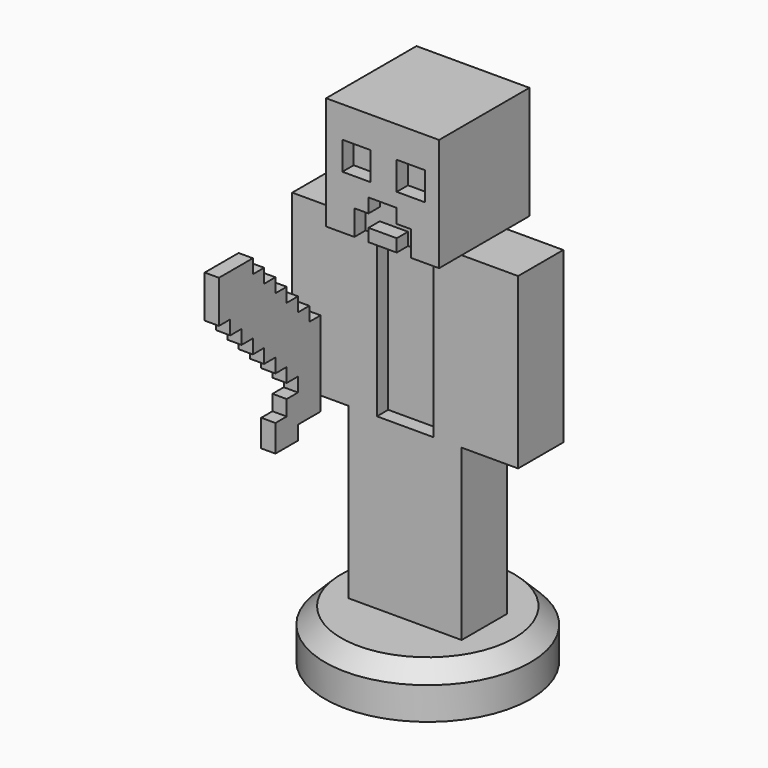
from build123d import *

# Parameters (mm, degrees)
F0_R      = 31.75
F1_DEPTH  = 15
F2_SIZE   = 5
F3_R      = 25
F4_DEPTH  = 10
F5_SIZE2  = 9.99999
F5_SIZE   = 24.99999
F6_W      = 34.925
F6_H      = 17.4625
F7_DEPTH  = 104.774
F10_W     = 34.925
F10_H     = 34.925
F11_DEPTH = 34.925
F12_W     = 17.4625
F12_H     = 17.4625
F13_DEPTH = 17.4625
F14_DEPTH = 34.925
F15_W     = 17.4625
F15_H     = 17.4625
F15_H_2   = 34.925
F16_DEPTH = 17.4625
F19_W     = 8.73125
F19_H     = 8.73125
F20_DEPTH = 4.365625
F17_W     = 4.365625
F17_H     = 4.365625
F23_DEPTH = 4.365625
F24_DEPTH = 4.365625
F25_W     = 4.4006995887
F25_H     = 4.365625
F26_DEPTH = 4.365625
F27_DEPTH = 8.73125
F28_W     = 4.4006995887
F28_H     = 4.365625
F29_DEPTH = 4.365625
F30_W     = 4.4006995887
F30_H     = 4.365625
F31_DEPTH = 4.365625
F32_W     = 4.4006995887
F32_H     = 4.365
F33_DEPTH = 4.365625
F34_DEPTH = 8.73125
F35_W     = 4.4006995887
F35_H     = 4.365
F36_DEPTH = 4.365625
F37_DEPTH = 8.73125
F38_W     = 4.4006995887
F38_H     = 4.365
F39_DEPTH = 4.365625
F40_DEPTH = 8.73125
F42_W     = 4.365625
F42_H     = 4.365625
F43_DEPTH = 4.365625
F44_DEPTH = 4.365625
F46_DEPTH = 8.73125
F47_W     = 4.365625
F47_H     = 4.365625
F48_DEPTH = 25
F41_W     = 4.4006995887
F41_H     = 4.365
F49_DEPTH = 4.365625
F50_DEPTH = 8.73125
F51_W     = 4.4006995887
F51_H     = 4.365
F52_DEPTH = 4.365625
F53_DEPTH = 8.73215
F54_W     = 4.4006995887
F54_H     = 4.3659
F55_DEPTH = 4.365625
F56_DEPTH = 4.365625
F57_W     = 4.4006995887
F57_H     = 4.365625
F58_DEPTH = 4.365625
F59_W     = 4.4006995887
F59_H     = 8.73125
F60_DEPTH = 4.365625
F61_DEPTH = 4.365625
F62_DEPTH = 4.365625
F63_DEPTH = 4.365625
F64_W     = 4.4006995887
F64_H     = 8.73125
F65_DEPTH = 4.365625
F66_W     = 4.4006995887
F66_H     = 4.36625
F66_H_2   = 4.365625
F67_DEPTH = 4.365625
F68_W     = 4.4006995887
F68_H     = 4.365625
F69_DEPTH = 4.365625
F70_W     = 4.4006995887
F70_H     = 4.4238492846
F70_H_2   = 3.9164990911
F71_DEPTH = 4.3565625
F21_W     = 17.4625
F21_H     = 52.3875
F72_DEPTH = 4.365625


# Not quite as in the source:
# - a fillet or chamfer is up to 0.001 mm smaller than in the source, because OpenCascade refuses the exact size


with BuildPart() as f1:
    # F0 (on Top) → F1 (new body)
    with BuildSketch(Plane.XY):
        Circle(F0_R)
    extrude(amount=F1_DEPTH)

    # F2
    f2_edges = [f1.edges().sort_by_distance(p)[0] for p in [
        (-31.75, 0, 15),
    ]]
    chamfer(f2_edges, length=F2_SIZE)

    # F3 (on face) → F4 (cut)
    with BuildSketch(Plane(origin=(0, 0, 0), x_dir=(1, 0, 0), z_dir=(0, 0, -1))):
        Circle(F3_R)
    extrude(amount=-F4_DEPTH, mode=Mode.SUBTRACT)

    # F5 (size 25 and 10 in the source; OpenCascade refuses exactly that, so slightly less here)
    f5_edges = [f1.edges().sort_by_distance(p)[0] for p in [
        (-25, 0, 10),
    ]]
    f5_side = f1.faces().sort_by_distance((0, 0, 10))[0]
    chamfer(f5_edges, length=F5_SIZE, length2=F5_SIZE2, reference=f5_side)

    # F6 (on face) → F7 (join)
    with BuildSketch(Plane.XY.offset(15)):
        Rectangle(F6_W, F6_H)
    extrude(amount=F7_DEPTH)

    # F10 (on face) → F11 (join)
    with BuildSketch(Plane.XY.offset(119.774)):
        Rectangle(F10_W, F10_H)
    extrude(amount=F11_DEPTH)

    # F12 (on face) → F13 (join)
    with BuildSketch(Plane.YZ.offset(17.4625)):
        with Locations((0, 111.04275)):
            Rectangle(F12_W, F12_H)
    extrude(amount=F13_DEPTH)

    # F14 (add): a face of the model
    f14_faces = [f1.faces().sort_by_distance(p)[0] for p in [
        (26.19375, 0, 102.3115),
    ]]
    extrude(f14_faces, amount=F14_DEPTH)

    # F15 (on face) → F16 (join)
    with BuildSketch(Plane(origin=(-17.4625, 0, 0), x_dir=(0, -1, 0), z_dir=(-1, 0, 0))):
        with Locations((0, 111.04275)):
            Rectangle(F15_W, F15_H)
        with Locations((0, 84.849)):
            Rectangle(F15_W, F15_H_2)
    extrude(amount=F16_DEPTH)

    # F19 (on face) → F20 (cut)
    with BuildSketch(Plane.XZ.offset(17.4625)):
        Polygon((-8.73125, 127.5853067636), (-8.73125, 119.774), (-4.365625, 119.774), (-4.365625, 123.6796533818), (4.365625, 123.6796533818), (4.365625, 119.774), (8.73125, 119.774), (8.73125, 127.5853067636), (4.365625, 127.5853067636), (4.365625, 131.9509317636), (-4.365625, 131.9509317636), (-4.365625, 127.5853067636), align=None)
        with Locations((-8.068405883, 140.6821817636)):
            Rectangle(F19_W, F19_H)
        with Locations((8.73125, 140.6821817636)):
            Rectangle(F19_W, F19_H)
    extrude(amount=-F20_DEPTH, mode=Mode.SUBTRACT)

    # F17 (on face) → F23 (join)
    with BuildSketch(Plane(origin=(0, 8.73125, 0), x_dir=(-1, 0, 0), z_dir=(0, 1, 0))):
        with Locations((28.3765625, 69.5693125)):
            Rectangle(F17_W, F17_H)
    extrude(amount=F23_DEPTH)

    # F24 (add): a face of the model
    f24_faces = [f1.faces().sort_by_distance(p)[0] for p in [
        (-28.3765625, 10.9140625, 71.752125),
    ]]
    extrude(f24_faces, amount=F24_DEPTH)

    # F25 (on face) → F26 (join)
    with BuildSketch(Plane.XZ.offset(8.73125)):
        with Locations((-28.3590252057, 69.5693125)):
            Rectangle(F25_W, F25_H)
    extrude(amount=F26_DEPTH)

    # F27 (add): a face of the model
    f27_faces = [f1.faces().sort_by_distance(p)[0] for p in [
        (-28.3590252057, -10.9140625, 71.752125),
    ]]
    extrude(f27_faces, amount=F27_DEPTH)

    # F28 (on face) → F29 (join)
    with BuildSketch(Plane.XZ.offset(13.096875)):
        with Locations((-28.3590252057, 73.9349375)):
            Rectangle(F28_W, F28_H)
        with Locations((-28.3590252057, 78.3005625)):
            Rectangle(F28_W, F28_H)
    extrude(amount=F29_DEPTH)

    # F30 (on face) → F31 (join)
    with BuildSketch(Plane.XY.offset(80.483375)):
        with Locations((-28.3590252057, -15.2796875)):
            Rectangle(F30_W, F30_H)
    extrude(amount=F31_DEPTH)

    # F32 (on face) → F33 (join)
    with BuildSketch(Plane.XZ.offset(17.4625)):
        with Locations((-28.3590252057, 78.300875)):
            Rectangle(F32_W, F32_H)
    extrude(amount=F33_DEPTH)

    # F34 (add): a face of the model
    f34_faces = [f1.faces().sort_by_distance(p)[0] for p in [
        (-28.3590252057, -19.6453125, 80.483375),
    ]]
    extrude(f34_faces, amount=F34_DEPTH)

    # F35 (on face) → F36 (join)
    with BuildSketch(Plane.XZ.offset(21.828125)):
        with Locations((-28.3590252057, 82.6665)):
            Rectangle(F35_W, F35_H)
    extrude(amount=F36_DEPTH)

    # F37 (add): a face of the model
    f37_faces = [f1.faces().sort_by_distance(p)[0] for p in [
        (-28.3590252057, -24.0109375, 84.849),
    ]]
    extrude(f37_faces, amount=F37_DEPTH)

    # F38 (on face) → F39 (join)
    with BuildSketch(Plane.XZ.offset(26.19375)):
        with Locations((-28.3590252057, 87.032125)):
            Rectangle(F38_W, F38_H)
    extrude(amount=F39_DEPTH)

    # F40 (add): a face of the model
    f40_faces = [f1.faces().sort_by_distance(p)[0] for p in [
        (-28.3590252057, -28.3765625, 89.214625),
    ]]
    extrude(f40_faces, amount=F40_DEPTH)

    # F42 (on face) → F43 (cut)
    with BuildSketch(Plane(origin=(0, 13.096875, 0), x_dir=(-1, 0, 0), z_dir=(0, 1, 0))):
        with Locations((28.3765625, 73.9349375)):
            Rectangle(F42_W, F42_H)
    extrude(amount=-F43_DEPTH, mode=Mode.SUBTRACT)

    # F44 (add): a face of the model
    f44_faces = [f1.faces().sort_by_distance(p)[0] for p in [
        (-28.3765625, 13.096875, 69.5693125),
    ]]
    extrude(f44_faces, amount=F44_DEPTH)

    # F45 (on face) → F46 (join)
    with BuildSketch(Plane(origin=(0, 0, 67.3865), x_dir=(1, 0, 0), z_dir=(0, 0, -1))):
        Polygon((-30.559375, -4.365625), (-30.559375, -8.73125), (-30.559375, -17.4625), (-26.19375, -17.4625), (-26.19375, -8.73125), (-26.19375, -4.365625), align=None)
    extrude(amount=F46_DEPTH)

    # F47 (on face) → F48 (cut)
    with BuildSketch(Plane(origin=(-30.559375, 0, 0), x_dir=(0, -1, 0), z_dir=(-1, 0, 0))):
        with Locations((-10.9140625, 65.2036875)):
            Rectangle(F47_W, F47_H)
    extrude(amount=-F48_DEPTH, mode=Mode.SUBTRACT)

    # F41 (on face) → F49 (join)
    with BuildSketch(Plane.XZ.offset(30.559375)):
        with Locations((-28.3590252057, 91.39775)):
            Rectangle(F41_W, F41_H)
    extrude(amount=F49_DEPTH)

    # F50 (add): a face of the model
    f50_faces = [f1.faces().sort_by_distance(p)[0] for p in [
        (-28.3590252057, -32.7421875, 93.58025),
    ]]
    extrude(f50_faces, amount=F50_DEPTH)

    # F51 (on face) → F52 (join)
    with BuildSketch(Plane.XZ.offset(34.925)):
        with Locations((-28.3590252057, 95.763375)):
            Rectangle(F51_W, F51_H)
    extrude(amount=F52_DEPTH)

    # F53 (add): a face of the model
    f53_faces = [f1.faces().sort_by_distance(p)[0] for p in [
        (-28.3590252057, -37.1078125, 97.945875),
    ]]
    extrude(f53_faces, amount=F53_DEPTH)

    # F54 (on face) → F55 (join)
    with BuildSketch(Plane.XZ.offset(39.290625)):
        with Locations((-28.3590252057, 100.12945)):
            Rectangle(F54_W, F54_H)
    extrude(amount=F55_DEPTH)

    # F56 (add): a face of the model
    f56_faces = [f1.faces().sort_by_distance(p)[0] for p in [
        (-28.3590252057, -41.4734375, 102.3124),
    ]]
    extrude(f56_faces, amount=F56_DEPTH)

    # F57 (on face) → F58 (join)
    with BuildSketch(Plane.XZ.offset(43.65625)):
        with Locations((-28.3590252057, 104.4952125)):
            Rectangle(F57_W, F57_H)
    extrude(amount=F58_DEPTH)

    # F59 (on face) → F60 (join)
    with BuildSketch(Plane.XY.offset(106.678025)):
        with Locations((-28.3590252057, -43.65625)):
            Rectangle(F59_W, F59_H)
    extrude(amount=F60_DEPTH)

    # F61 (add): faces of the model
    f61_faces = [f1.faces().sort_by_distance(p)[0] for p in [
        (-28.3590252057, -10.9140625, 80.483375),
        (-28.3590252057, -15.2796875, 84.849),
        (-28.3590252057, -19.6453125, 89.214625),
        (-28.3590252057, -24.0109375, 93.58025),
        (-28.3590252057, -28.3765625, 97.945875),
        (-28.3590252057, -32.7421875, 102.3115),
        (-28.3590252057, -37.1078125, 106.678025),
        (-28.3590252057, -43.65625, 111.04365),
    ]]
    extrude(f61_faces, amount=F61_DEPTH)

    # F62 (add): faces of the model
    f62_faces = [f1.faces().sort_by_distance(p)[0] for p in [
        (-28.3590252057, -10.9140625, 84.849),
        (-28.3590252057, -15.2796875, 89.214625),
        (-28.3590252057, -19.6453125, 93.58025),
        (-28.3590252057, -24.0109375, 97.945875),
        (-28.3590252057, -28.3765625, 102.3115),
        (-28.3590252057, -32.7421875, 106.677125),
        (-28.3590252057, -37.1078125, 111.04365),
    ]]
    extrude(f62_faces, amount=F62_DEPTH)

    # F63 (add): a face of the model
    f63_faces = [f1.faces().sort_by_distance(p)[0] for p in [
        (-28.3590252057, -15.2796875, 71.752125),
    ]]
    extrude(f63_faces, amount=F63_DEPTH)

    # F64 (on face) → F65 (join)
    with BuildSketch(Plane(origin=(0, 0, 67.3865), x_dir=(1, 0, 0), z_dir=(0, 0, -1))):
        with Locations((-28.3590252057, 13.096875)):
            Rectangle(F64_W, F64_H)
    extrude(amount=F65_DEPTH)

    # F66 (on face) → F67 (join)
    with BuildSketch(Plane.XZ.offset(17.4625)):
        with Locations((-28.3590252057, 69.569625)):
            Rectangle(F66_W, F66_H)
        with Locations((-28.3590252057, 65.2036875)):
            Rectangle(F66_W, F66_H_2)
    extrude(amount=F67_DEPTH)

    # F68 (on face) → F69 (join)
    with BuildSketch(Plane(origin=(0, 0, 63.020875), x_dir=(1, 0, 0), z_dir=(0, 0, -1))):
        with Locations((-28.3590252057, 19.6453125)):
            Rectangle(F68_W, F68_H)
    extrude(amount=F69_DEPTH)

    # F70 (on face) → F71 (join)
    with BuildSketch(Plane.XZ.offset(21.828125)):
        with Locations((-28.3590252057, 64.7836737335)):
            Rectangle(F70_W, F70_H)
        with Locations((-28.3590252057, 60.6134995456)):
            Rectangle(F70_W, F70_H_2)
    extrude(amount=F71_DEPTH)

    # F21 (on face) → F72 (cut)
    with BuildSketch(Plane.XZ.offset(8.73125)):
        with Locations((0, 93.58025)):
            Rectangle(F21_W, F21_H)
    extrude(amount=-F72_DEPTH, mode=Mode.SUBTRACT)


solid = f1.part
